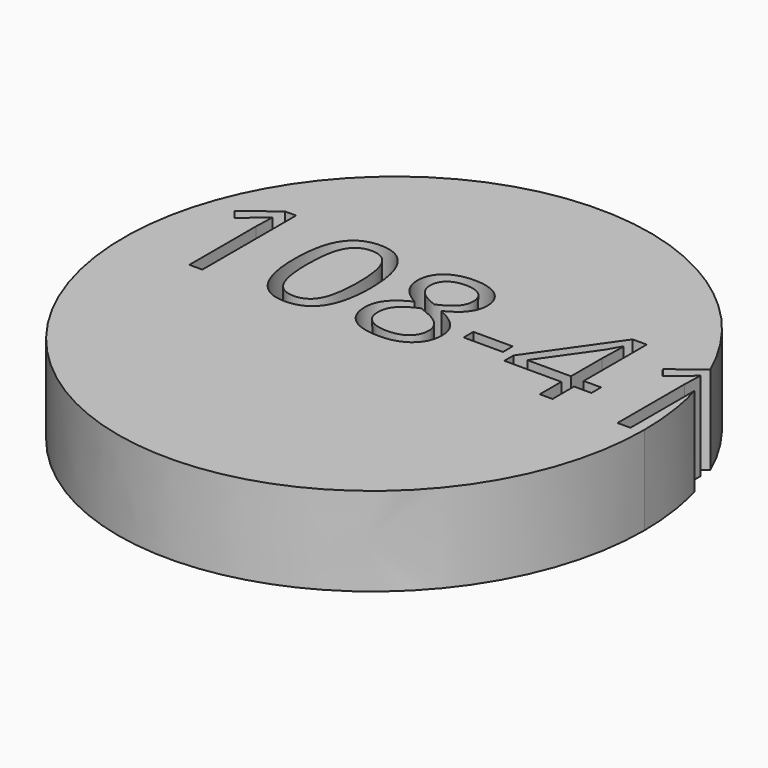
from build123d import *

# Parameters (mm, degrees)
F1_DEPTH     = 25.4
F2_TEXT_SIZE = 47.0644000267
F3_DEPTH     = 25.4


# Not quite as in the source:
# - Text() gives the source's letters only with a copy of the font that has no kerning and outlines rounded to 1/6400 em; it was checked with that copy


with BuildPart() as f1:
    # F0 (on Top) → F1 (new body)
    with BuildSketch(Plane.XY):
        with BuildLine():
            add(Edge.make_bspline(
                [(74.6471434832, 0), (74.6471434832, 133.824328695), (-37.3235717416, 66.9121643475), (-149.2942869663, 0), (-37.3235717416, -66.9121643475), (74.6471434832, -133.824328695), (74.6471434832, 0)],
                knots=[4.7123889804, 4.7123889804, 4.7123889804, 6.8067840828, 6.8067840828, 8.9011791852, 8.9011791852, 10.9955742876, 10.9955742876, 10.9955742876], degree=2, weights=[1, 0.5, 1, 0.5, 1, 0.5, 1]))
        make_face()
    extrude(amount=F1_DEPTH)

    # F2 (on face) → F3 (cut)
    with BuildSketch(Plane.XY.offset(25.4)):
        with Locations((-67.6131964996, -1.144555354)):
            Text('108-41', F2_TEXT_SIZE, font='Open Sans', text_align=(TextAlign.LEFT, TextAlign.BOTTOM))
    extrude(amount=-F3_DEPTH, mode=Mode.SUBTRACT)


solid = f1.part
